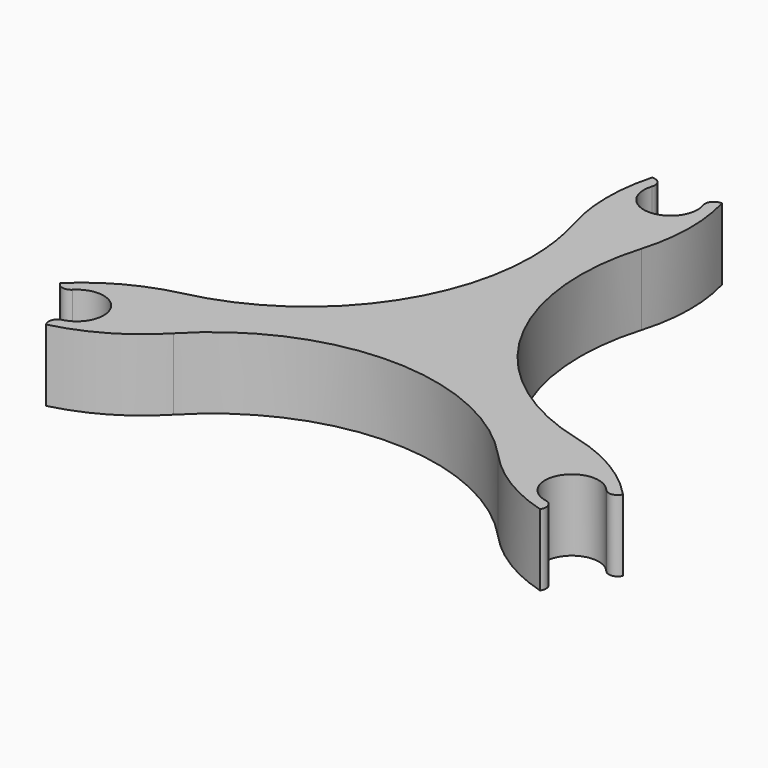
from build123d import *

# Parameters (mm, degrees)
F1_DEPTH    = 8
F2_R        = 1
F3_T1_DEPTH = 64.2226111809
F3_T3_DEPTH = 65.5041643561
F3_T5_DEPTH = 66.9229315715
F3_T7_DEPTH = 64.2892221554
F3_T9_DEPTH = 66.1623607225


# Not quite as in the source:
# - a fillet or chamfer that OpenCascade refuses, or shapes differently, is made with other operations: its cross-section is extruded or revolved along the edge and cut away or added


with BuildPart() as f1:
    # F0 (on Top) → F1 (new body)
    with BuildSketch(Plane.XY):
        with BuildLine():
            ThreePointArc((1.7213359453, 34.45703125), (0, 29), (-1.7213359453, 34.45703125))
            ThreePointArc((-1.7213359453, 34.45703125), (-5.6630518779, 34.0320414232), (-9.5299848811, 33.1576444906))
            ThreePointArc((-9.5299848811, 33.1576444906), (-4.4795318248, 25.2311781209), (-2.7128129211, 16))
            ThreePointArc((-2.7128129211, 16), (-12.2077903389, -3.6110753077), (-33.4803548991, -8.3256132406))
            ThreePointArc((-33.4803548991, -8.3256132406), (-32.3848639744, -11.8941407997), (-30.9102371196, -15.3234213285))
            ThreePointArc((-30.9102371196, -15.3234213285), (-25.3652162283, -14.4450583373), (-28.9498248331, -18.7658637459))
            ThreePointArc((-28.9498248331, -18.7658637459), (-26.6234342426, -21.9418036891), (-23.950370018, -24.83203125))
            ThreePointArc((-23.950370018, -24.83203125), (0, -7), (23.950370018, -24.83203125))
            ThreePointArc((23.950370018, -24.83203125), (26.587584538, -21.9852302339), (28.8884099574, -18.8602696198))
            ThreePointArc((28.8884099574, -18.8602696198), (24.9364218636, -14.6683482508), (30.5204410338, -16.0857912178))
            ThreePointArc((30.5204410338, -16.0857912178), (32.2347725379, -12.2950981871), (33.4803548991, -8.3256132406))
            ThreePointArc((33.4803548991, -8.3256132406), (6.0621778265, 3.5), (9.5299848811, 33.1576444906))
            ThreePointArc((9.5299848811, 33.1576444906), (5.6630518779, 34.0320414232), (1.7213359453, 34.45703125))
        make_face()
    extrude(amount=F1_DEPTH)

    # F2
    f2_edges = [f1.edges().sort_by_distance(p)[0] for p in [
        (-30.910237, -15.323421, 4),
        (-28.949825, -18.765864, 4),
        (1.721336, 34.457031, 4),
        (-1.721336, 34.457031, 4),
        (28.88841, -18.86027, 4),
        (30.520441, -16.085791, 4),
    ]]
    fillet(f2_edges, radius=F2_R)

    # F3: fillet of radius 20 on 6 edges, made by hand

    # F3_s2 → F3_t1 (cut)
    with BuildSketch(Plane.XY.offset(-28.1113055904)):
        with BuildLine():
            ThreePointArc((-22.2360329208, -8.3927218823), (-27.3415731158, -10.3001532277), (-31.7425915451, -13.5150982979))
            ThreePointArc((-31.7425915451, -13.5150982979), (-32.7145361346, -10.9548676622), (-33.4803548991, -8.3256132406))
            ThreePointArc((-33.4803548991, -8.3256132406), (-27.8620158848, -8.9995547655), (-22.2360329208, -8.3927218823))
        make_face()
    extrude(amount=F3_T1_DEPTH, mode=Mode.SUBTRACT)

    # F3_s4 → F3_t3 (cut)
    with BuildSketch(Plane.XY.offset(-28.7520821781)):
        with BuildLine():
            ThreePointArc((-3.9009970628, 34.2787430037), (-4.619010619, 28.731142286), (-3.7725584788, 23.2016815561))
            ThreePointArc((-3.7725584788, 23.2016815561), (-6.0709826163, 28.5152379545), (-9.5299848811, 33.1576444906))
            ThreePointArc((-9.5299848811, 33.1576444906), (-6.7388451877, 33.8354542682), (-3.9009970628, 34.2787430037))
        make_face()
        with BuildLine():
            ThreePointArc((3.9009970628, 34.2787430037), (4.619010619, 28.731142286), (3.7725584788, 23.2016815561))
            ThreePointArc((3.7725584788, 23.2016815561), (6.0709826163, 28.5152379545), (9.5299848811, 33.1576444906))
            ThreePointArc((9.5299848811, 33.1576444906), (6.7388451877, 33.8354542682), (3.9009970628, 34.2787430037))
        make_face()
    extrude(amount=F3_T3_DEPTH, mode=Mode.SUBTRACT)

    # F3_s6 → F3_t5 (cut)
    with BuildSketch(Plane.XY.offset(-29.4614657857)):
        with BuildLine():
            ThreePointArc((21.695923744, -8.2651405236), (27.0245333746, -10.4395796023), (31.513317936, -14.0413956808))
            ThreePointArc((31.513317936, -14.0413956808), (32.6222611015, -11.2266682781), (33.4803548991, -8.3256132406))
            ThreePointArc((33.4803548991, -8.3256132406), (27.5845251828, -8.999670843), (21.695923744, -8.2651405236))
        make_face()
    extrude(amount=F3_T5_DEPTH, mode=Mode.SUBTRACT)

    # F3_s8 → F3_t7 (cut)
    with BuildSketch(Plane.XY.offset(-28.1446110777)):
        with BuildLine():
            ThreePointArc((27.5839500196, -20.7213827076), (22.5899865116, -18.5199962805), (18.3770596718, -15.0505552356))
            ThreePointArc((18.3770596718, -15.0505552356), (21.7214673604, -19.6234958203), (23.950370018, -24.83203125))
            ThreePointArc((23.950370018, -24.83203125), (25.8490017853, -22.8490504552), (27.5839500196, -20.7213827076))
        make_face()
    extrude(amount=F3_T7_DEPTH, mode=Mode.SUBTRACT)

    # F3_s10 → F3_t9 (cut)
    with BuildSketch(Plane.XY.offset(-29.0811803612)):
        with BuildLine():
            ThreePointArc((-18.1139750308, -14.7696805432), (-22.5633062196, -18.281704114), (-27.8192704457, -20.4043669804))
            ThreePointArc((-27.8192704457, -20.4043669804), (-25.9793181426, -22.7007715474), (-23.950370018, -24.83203125))
            ThreePointArc((-23.950370018, -24.83203125), (-21.6255637275, -19.4566753424), (-18.1139750308, -14.7696805432))
        make_face()
    extrude(amount=F3_T9_DEPTH, mode=Mode.SUBTRACT)


solid = f1.part
